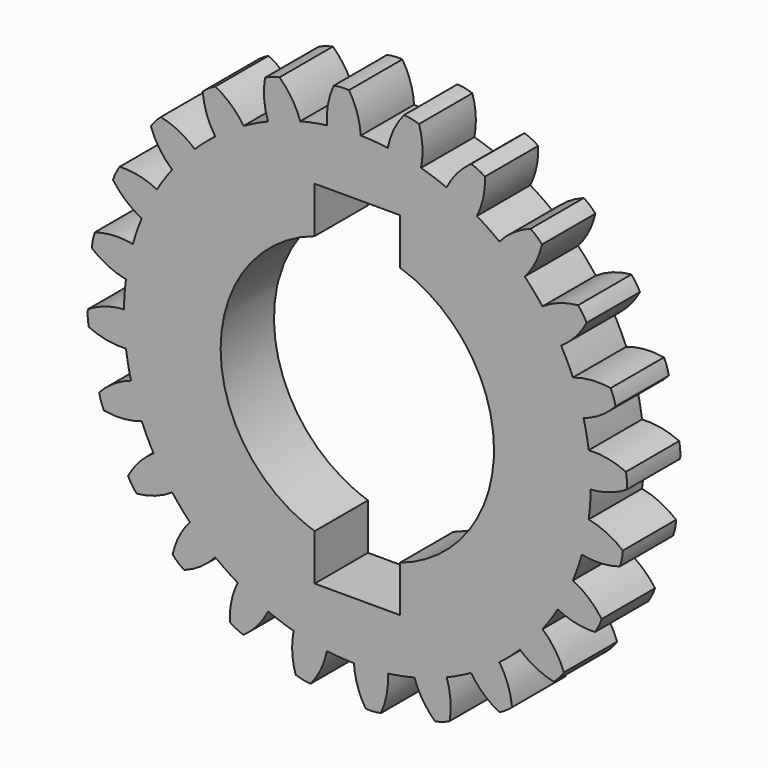
from build123d import *

# Parameters (mm, degrees)
F1_DEPTH = 12.7
F2_COUNT = 24
F2_ANGLE = 345
F3_DEPTH = 25.4


# Not quite as in the source:
# - a feature names something its author has since deleted; it is built from what else it names


with BuildPart() as f1:
    # F0 (on Front) → F1 (new body)
    with BuildSketch(Plane.XZ):
        with BuildLine():
            ThreePointArc((-5.81118052, 44.0684998719), (-29.3043983549, -33.4223688128), (44.45, 0))
            ThreePointArc((44.45, 0), (31.6596085179, 31.2005078243), (0.6492491116, 44.4452581902))
            ThreePointArc((0.6492491116, 44.4452581902), (-2.5878312685, 44.3746056808), (-5.81118052, 44.0684998719))
        make_face()
        with BuildLine():
            ThreePointArc((8.128, 24.7337187054), (21.0883108024, 15.2677559746), (26.035, 0))
            ThreePointArc((26.035, 0), (21.0883108024, -15.2677559746), (8.128, -24.7337187054))
            Line((8.128, -24.7337187054), (8.128, -33.528))
            Line((8.128, -33.528), (-8.128, -33.528))
            Line((-8.128, -33.528), (-8.128, -24.7337187054))
            ThreePointArc((-8.128, -24.7337187054), (-26.035, 0), (-8.128, 24.7337187054))
            Line((-8.128, 24.7337187054), (-8.128, 33.528))
            Line((-8.128, 33.528), (8.128, 33.528))
            Line((8.128, 33.528), (8.128, 24.7337187054))
        make_face(mode=Mode.SUBTRACT)
        with BuildLine():
            ThreePointArc((-5.81118052, 44.0684998719), (-2.5878312685, 44.3746056808), (0.6492491116, 44.4452581902))
            ThreePointArc((0.6492491116, 44.4452581902), (-0.0343594341, 48.0324601777), (-1.5864878253, 51.3379459514))
            ThreePointArc((-1.5864878253, 51.3379459514), (-3.0455527066, 51.3454237754), (-4.4911590337, 51.147563742))
            ThreePointArc((-4.4911590337, 51.147563742), (-5.5943052126, 47.6906625485), (-5.81118052, 44.0684998719))
        make_face()
    extrude(amount=F1_DEPTH)

    # F2: F1 ×24 about axis
    f2_axis = Axis((0, 0, 0), (0, 1, 0))


with BuildPart() as f1_1:
    add(f1.part)
    for i in range(1, F2_COUNT):
        add(f1.part.rotate(f2_axis, i * F2_ANGLE / (F2_COUNT - 1)))


with BuildPart() as f3:
    # F0 (on Front) → F3 (new body, symmetric)
    with BuildSketch(Plane.XZ):
        with BuildLine():
            ThreePointArc((-8.128, 24.7337187054), (0, 26.035), (8.128, 24.7337187054))
            Line((8.128, 24.7337187054), (8.128, 33.528))
            Line((8.128, 33.528), (-8.128, 33.528))
            Line((-8.128, 33.528), (-8.128, 24.7337187054))
        make_face()
    extrude(amount=F3_DEPTH, both=True)


with BuildPart() as f3b:
    # F0 (on Front) → F3, piece 2 (new body, symmetric)
    with BuildSketch(Plane.XZ):
        with BuildLine():
            Line((8.128, -33.528), (8.128, -24.7337187054))
            ThreePointArc((8.128, -24.7337187054), (0, -26.035), (-8.128, -24.7337187054))
            Line((-8.128, -24.7337187054), (-8.128, -33.528))
            Line((-8.128, -33.528), (8.128, -33.528))
        make_face()
    extrude(amount=F3_DEPTH, both=True)


with BuildPart() as f1_2:
    add(f1_1.part)

    # F4: cut F3, F3b
    add(f3.part, mode=Mode.SUBTRACT)
    add(f3b.part, mode=Mode.SUBTRACT)


solid = f1_2.part
